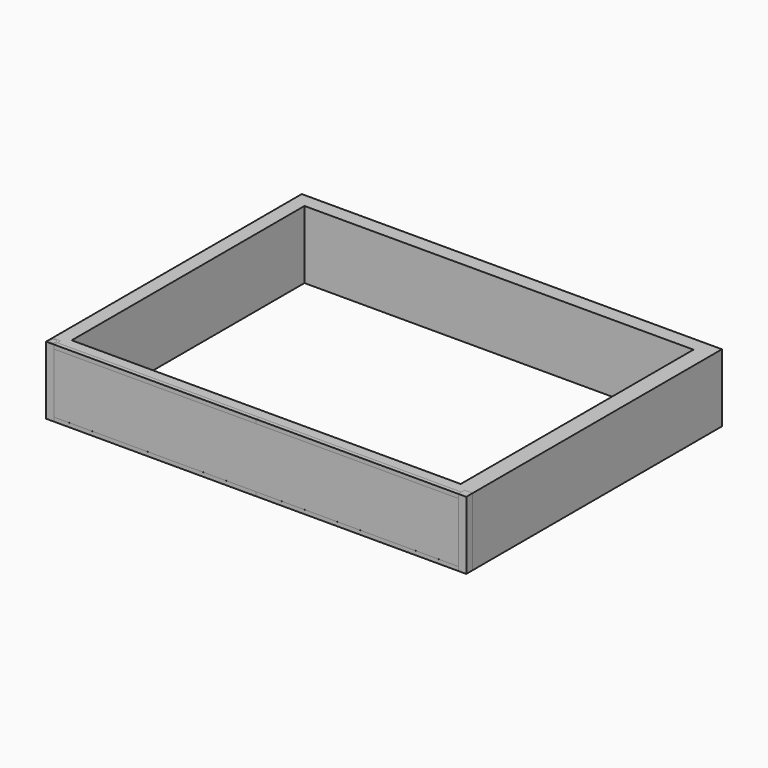
from build123d import *

# Parameters (mm, degrees)
F0_W          = 501.3666492069
F0_H          = 381.3144250231
F0_W_2        = 464.144741692
F0_H_2        = 347.1421356561
F1_DEPTH      = 81
F2_W          = 9.525
F2_H          = 9.525
F3_DEPTH      = 81.01
F3_DEPTH_BACK = 0.01
F4_W          = 241.1683246034
F4_H          = 4.7625
F5_DEPTH      = 4.7625
F11_R         = 3.175
F12_DEPTH     = 14


# Not quite as in the source:
# - a length typed as a fraction of an inch, garbled in the dataset ("3 / 203.2 mm" for 3/8 in), is restored


with BuildPart() as f1:
    # F0 (on Top) → F1 (new body)
    with BuildSketch(Plane.XY):
        with Locations((250.6833246034, 190.6572125116)):
            Rectangle(F0_W, F0_H)
        with Locations((249.072370846, 190.5710678281)):
            Rectangle(F0_W_2, F0_H_2, mode=Mode.SUBTRACT)
    extrude(amount=F1_DEPTH)


with BuildPart() as f3:
    # F2 (on Top) → F3 (new body, two sides)
    with BuildSketch(Plane.XY) as f3_sk:
        with Locations((4.7525, 4.7525)):
            Rectangle(F2_W, F2_H)
    extrude(amount=F3_DEPTH)
    extrude(f3_sk.sketch, amount=-F3_DEPTH_BACK)


with BuildPart() as f5:
    # F4 (on face) → F5 (new body)
    with BuildSketch(Plane.XZ.offset(0.01)):
        with Locations((130.0991623017, 2.37125)):
            Rectangle(F4_W, F4_H)
    extrude(amount=-F5_DEPTH)


with BuildPart() as f9_1:
    # F9: instance of F3
    add(f3.part.mirror(Plane.YZ.offset(250.6833246034)))


with BuildPart() as f9_2:
    # F9: instance of F5
    add(f5.part.mirror(Plane.YZ.offset(250.6833246034)))


with BuildPart() as f10_1:
    # F10: instance of F9_2
    add(f9_2.part.mirror(Plane.XY.offset(40.5)))


with BuildPart() as f10_2:
    # F10: instance of F5
    add(f5.part.mirror(Plane.XY.offset(40.5)))


with BuildPart() as f3_1:
    add(f3.part)

    # F11 (on face) → F12 (cut)
    with BuildSketch(Plane.XY.offset(81.01)):
        with Locations((4.7575, 4.7575)):
            Circle(F11_R)
    extrude(amount=-F12_DEPTH, mode=Mode.SUBTRACT)


solid = Compound([f1.part, f5.part, f9_1.part, f9_2.part, f10_1.part, f10_2.part, f3_1.part])
